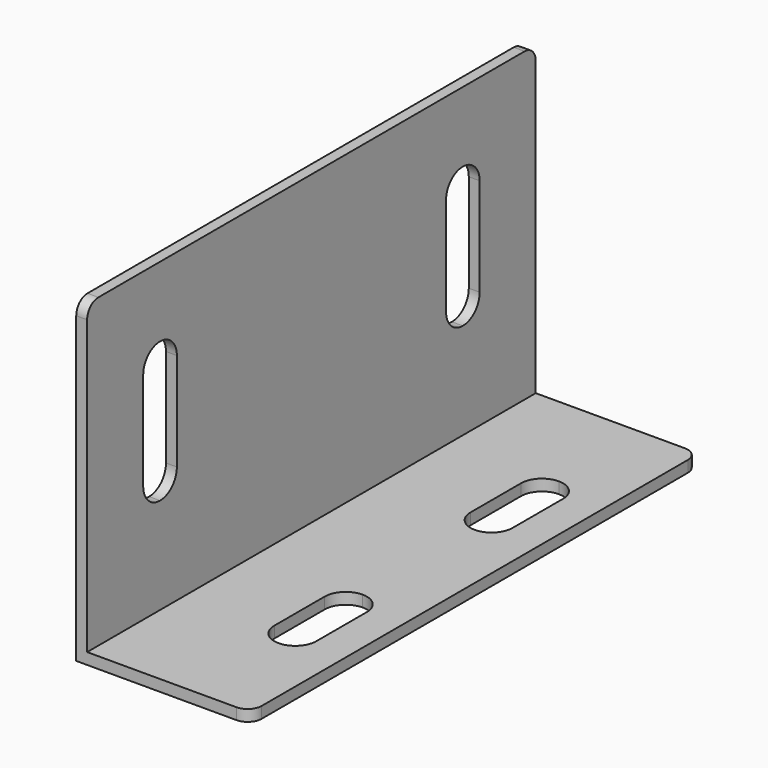
from build123d import *

# Parameters (mm, degrees)
F1_DEPTH = 203.2
F2_R     = 5.08
F3_W     = 15.24
F3_H     = 50.8
F4_DEPTH = 3.9456780069
F5_R     = 7.61999
F6_W     = 15.24
F6_H     = 38.1
F7_DEPTH = 4.1115754284
F8_R     = 7.61999


# Not quite as in the source:
# - a fillet or chamfer is up to 0.001 mm smaller than in the source, because OpenCascade refuses the exact size


with BuildPart() as f1:
    # F0 (on Front) → F1 (new body)
    with BuildSketch(Plane.XZ):
        Polygon((59.1770336032, 0), (0, 0), (0, 111.0939458013), (-3.9456780069, 111.0939458013), (-3.9456780069, -4.1115754284), (59.1770336032, -4.1115754284), align=None)
    extrude(amount=F1_DEPTH)

    # F2
    f2_edges = [f1.edges().sort_by_distance(p)[0] for p in [
        (-1.972839, -203.2, 111.093946),
        (59.177034, -203.2, -2.055788),
        (59.177034, 0, -2.055788),
        (-1.972839, 0, 111.093946),
    ]]
    fillet(f2_edges, radius=F2_R)

    # F3 (on face) → F4 (cut, through all)
    with BuildSketch(Plane.YZ):
        with Locations((-170.18, 60.2939458013)):
            Rectangle(F3_W, F3_H)
        with Locations((-33.02, 60.2939458013)):
            Rectangle(F3_W, F3_H)
    extrude(amount=-F4_DEPTH, mode=Mode.SUBTRACT)

    # F5 (radius 7.62 in the source; OpenCascade refuses exactly that, so slightly less here)
    f5_edges = [f1.edges().sort_by_distance(p)[0] for p in [
        (-1.972839, -177.8, 34.893946),
        (-1.972839, -162.56, 34.893946),
        (-1.972839, -177.8, 85.693946),
        (-1.972839, -162.56, 85.693946),
        (-1.972839, -40.64, 85.693946),
        (-1.972839, -25.4, 85.693946),
        (-1.972839, -40.64, 34.893946),
        (-1.972839, -25.4, 34.893946),
    ]]
    fillet(f5_edges, radius=F5_R)

    # F6 (on face) → F7 (cut, through all)
    with BuildSketch(Plane.XY):
        with Locations((38.8570336032, -146.05)):
            Rectangle(F6_W, F6_H)
        with Locations((38.8570336032, -57.15)):
            Rectangle(F6_W, F6_H)
    extrude(amount=-F7_DEPTH, mode=Mode.SUBTRACT)

    # F8 (radius 7.62 in the source; OpenCascade refuses exactly that, so slightly less here)
    f8_edges = [f1.edges().sort_by_distance(p)[0] for p in [
        (31.237034, -165.1, -2.055788),
        (46.477034, -165.1, -2.055788),
        (31.237034, -127, -2.055788),
        (46.477034, -127, -2.055788),
        (46.477034, -38.1, -2.055788),
        (46.477034, -76.2, -2.055788),
        (31.237034, -76.2, -2.055788),
        (31.237034, -38.1, -2.055788),
    ]]
    fillet(f8_edges, radius=F8_R)


solid = f1.part
